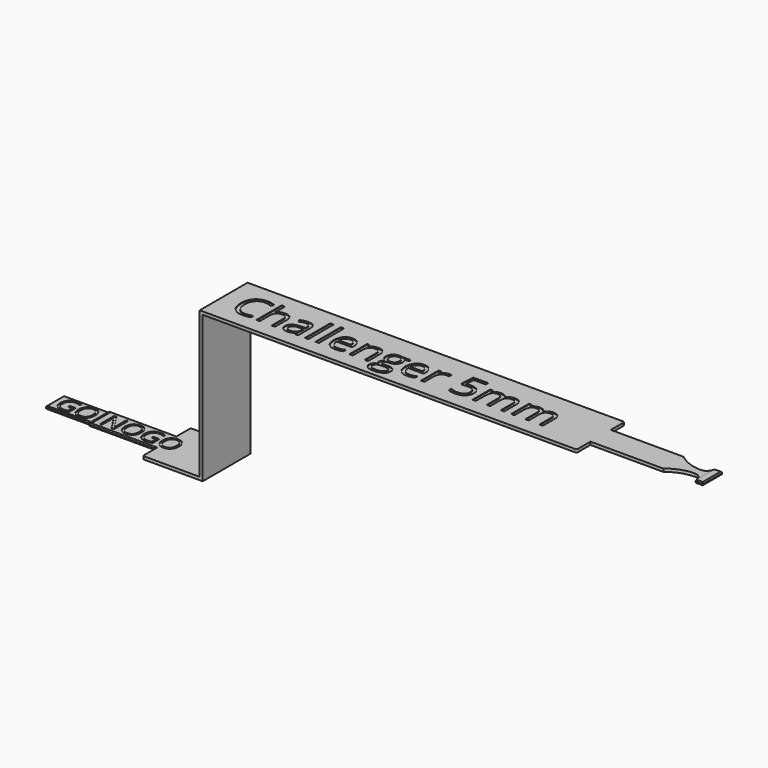
from build123d import *

# Parameters (mm, degrees)
F1_DEPTH      = 4
F0_W          = 9
F0_H          = 0.4
F2_DEPTH      = 1.75
F0_W_2        = 6
F3_DEPTH      = 1.55
F0_W_3        = 1
F4_DEPTH      = 1.65
F0_W_4        = 8
F5_DEPTH      = 1.7
F6_DEPTH      = 0.5
F8_DEPTH      = 0.4
F10_DEPTH     = 0.4
F11_SIZE      = 0.15
F11_2_SIZE    = 0.15
F12_R         = 0.2
F12_2_R       = 0.2
F13_TEXT_SIZE = 3.3333333333
F14_DEPTH     = 0.1
F15_TEXT_SIZE = 5.5555555556
F16_DEPTH     = 0.1
F17_DEPTH     = 0.4
F19_DEPTH     = 25


# Not quite as in the source:
# - a feature names something its author has since deleted; it is built from what else it names
# - Text() gives the source's letters only with a copy of the font that has no kerning and outlines rounded to 1/6400 em; it was checked with that copy


with BuildPart() as f1:
    # F0 (on Front) → F1 (new body, symmetric)
    with BuildSketch(Plane.XZ):
        Polygon((15, 0.4), (15, 0), (23, 0), (23, 19.6), (73, 19.6), (73, 20), (22.6, 20), (22.6, 0.4), align=None)
    extrude(amount=F1_DEPTH, both=True)

    # F0 (on Front) → F2 (join, symmetric)
    with BuildSketch(Plane.XZ):
        with Locations((10.5, 0.2)):
            Rectangle(F0_W, F0_H)
    extrude(amount=F2_DEPTH, both=True)

    # F0 (on Front) → F3 (join, symmetric)
    with BuildSketch(Plane.XZ):
        with Locations((3, 0.2)):
            Rectangle(F0_W_2, F0_H)
    extrude(amount=F3_DEPTH, both=True)

    # F0 (on Front) → F5 (join, symmetric)
    with BuildSketch(Plane.XZ):
        with Locations((77, 19.8)):
            Rectangle(F0_W_4, F0_H)
    extrude(amount=F5_DEPTH, both=True)

    # F0 (on Front) → F6 (join, symmetric)
    with BuildSketch(Plane.XZ):
        with Locations((84, 19.8)):
            Rectangle(F0_W_2, F0_H)
    extrude(amount=F6_DEPTH, both=True)

    # F7 (on face) → F8 (join)
    with BuildSketch(Plane.XY.offset(20)):
        with BuildLine():
            Line((87, 0.5), (87, 1.5))
            ThreePointArc((87, 1.5), (86.7071067812, 0.7928932188), (86, 0.5))
            Line((86, 0.5), (87, 0.5))
        make_face()
        with BuildLine():
            Line((87, -1.5), (87, -0.5))
            Line((87, -0.5), (86, -0.5))
            ThreePointArc((86, -0.5), (86.7071067812, -0.7928932188), (87, -1.5))
        make_face()
    extrude(amount=-F8_DEPTH)

    # F9 (on face) → F10 (join)
    with BuildSketch(Plane.XY.offset(20)):
        with BuildLine():
            Line((81, 0.5), (81, 1.7))
            Line((81, 1.7), (73, 1.7))
            Line((73, 1.7), (73, 4))
            Line((73, 4), (22.6, 4))
            Line((22.6, 4), (22.6, -4))
            Line((22.6, -4), (73, -4))
            Line((73, -4), (73, -1.7))
            Line((73, -1.7), (81, -1.7))
            Line((81, -1.7), (81, -0.5))
            Line((81, -0.5), (86, -0.5))
            ThreePointArc((86, -0.5), (86.7071067812, -0.7928932188), (87, -1.5))
            Line((87, -1.5), (87, 1.5))
            ThreePointArc((87, 1.5), (86.7071067812, 0.7928932188), (86, 0.5))
            Line((86, 0.5), (81, 0.5))
        make_face()
        with BuildLine():
            ThreePointArc((82.7503846381, -1.7), (84.2679491924, -0.8095842402), (86, -0.5))
            Line((86, -0.5), (81, -0.5))
            Line((81, -0.5), (81, -1.7))
            Line((81, -1.7), (82.7503846381, -1.7))
        make_face()
        with BuildLine():
            Line((82.7503846381, 1.7), (81, 1.7))
            Line((81, 1.7), (81, 0.5))
            Line((81, 0.5), (86, 0.5))
            ThreePointArc((86, 0.5), (84.2679491924, 0.8095842402), (82.7503846381, 1.7))
        make_face()
    extrude(amount=-F10_DEPTH)

    # F11
    f11_edges = [f1.edges().sort_by_distance(p)[0] for p in [
        (10.5, 1.75, 0.4),
        (10.5, 1.75, 0),
        (10.5, -1.75, 0.4),
        (10.5, -1.75, 0),
        (3, -1.55, 0.4),
        (3, -1.55, 0),
        (0, 0, 0.4),
        (0, 0, 0),
        (3, 1.55, 0.4),
        (3, 1.55, 0),
    ]]
    chamfer(f11_edges, length=F11_SIZE)

    # F12
    f12_edges = [f1.edges().sort_by_distance(p)[0] for p in [
        (73, -4, 19.8),
        (73, 4, 19.8),
        (15, 4, 0.2),
        (15, -4, 0.2),
        (0, 1.55, 0.2),
        (0, -1.55, 0.2),
    ]]
    fillet(f12_edges, radius=F12_R)

    # F13 (on face) → F14 (cut)
    with BuildSketch(Plane.XY.offset(0.4)):
        with Locations((0.6, -1.2)):
            Text('GO', F13_TEXT_SIZE, font='Open Sans', text_align=(TextAlign.LEFT, TextAlign.BOTTOM))
        with Locations((6.7, -1.2)):
            Text('NOGO', F13_TEXT_SIZE, font='Open Sans', text_align=(TextAlign.LEFT, TextAlign.BOTTOM))
        Polygon((6, -1.4), (6, -1.55), (6, -1.6), (6.2, -1.6), (6.2, 1.6), (6, 1.6), (6, 1.55), (6, 1.4), align=None)
    extrude(amount=-F14_DEPTH, mode=Mode.SUBTRACT)

    # F15 (on face) → F16 (cut)
    with BuildSketch(Plane.XY.offset(20)):
        with Locations((24.6, -2)):
            Text('Challenger 5mm', F15_TEXT_SIZE, font='Open Sans', text_align=(TextAlign.LEFT, TextAlign.BOTTOM))
    extrude(amount=-F16_DEPTH, mode=Mode.SUBTRACT)

    # F9 (on face) → F17 (join)
    with BuildSketch(Plane.XY.offset(20)):
        with BuildLine():
            Line((82.7503846381, 1.7), (81, 1.7))
            Line((81, 1.7), (81, 0.5))
            Line((81, 0.5), (86, 0.5))
            ThreePointArc((86, 0.5), (84.2679491924, 0.8095842402), (82.7503846381, 1.7))
        make_face()
    extrude(amount=-F17_DEPTH)

    # F18 (on Top) → F19 (cut)
    with BuildSketch(Plane.XY):
        Polygon((6, -1.55), (0, -1.5), (0, -1.55), align=None)
        Polygon((-0.0004166667, 1.55), (0, 1.5), (6, 1.55), align=None)
    extrude(amount=F19_DEPTH, mode=Mode.SUBTRACT)


with BuildPart() as f4:
    # F0 (on Front) → F4 (new body, symmetric)
    with BuildSketch(Plane.XZ):
        with Locations((87.5, 19.8)):
            Rectangle(F0_W_3, F0_H)
    extrude(amount=F4_DEPTH, both=True)

    # F11#2
    f11_2_edges = [f4.edges().sort_by_distance(p)[0] for p in [
        (88, 0, 20),
        (88, 0, 19.6),
        (87.5, -1.65, 20),
        (87.5, -1.65, 19.6),
        (87.5, 1.65, 20),
        (87.5, 1.65, 19.6),
    ]]
    chamfer(f11_2_edges, length=F11_2_SIZE)

    # F12#2
    f12_2_edges = [f4.edges().sort_by_distance(p)[0] for p in [
        (88, -1.65, 19.8),
        (88, 1.65, 19.8),
    ]]
    fillet(f12_2_edges, radius=F12_2_R)


solid = Compound([f1.part, f4.part])
